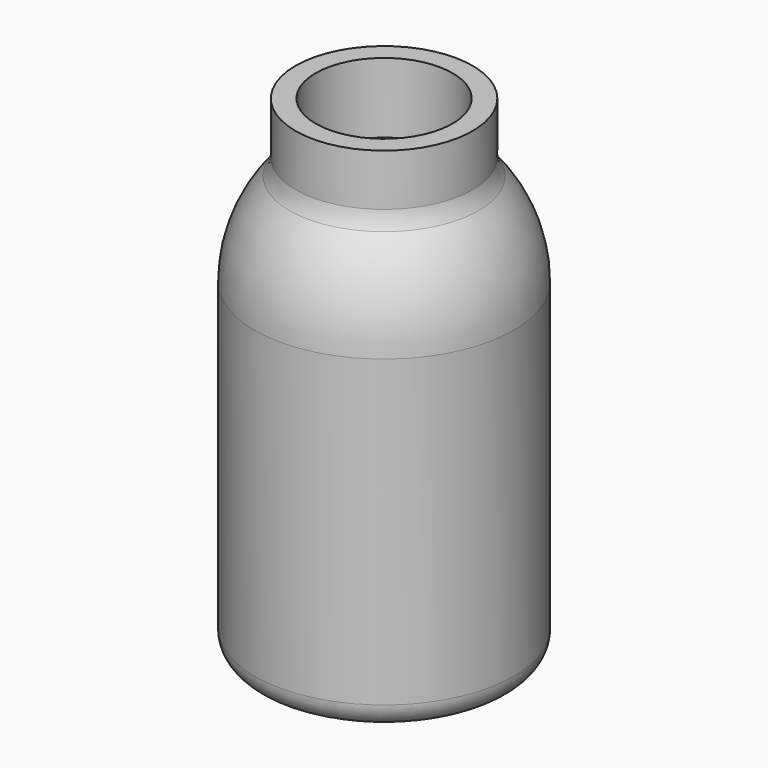
from build123d import *

# Parameters (mm, degrees)
F3_R = 5.08


# Not quite as in the source:
# - a fillet or chamfer that OpenCascade refuses, or shapes differently, is made with other operations: its cross-section is extruded or revolved along the edge and cut away or added


with BuildPart() as f1:
    # F0 (on Front) → F1 (revolve)
    with BuildSketch(Plane.XZ):
        with BuildLine():
            Line((-26.2792315334, 0), (-22.2152307564, 0))
            Line((-22.2152307564, 0), (-22.2152307564, 66.6416212916))
            ThreePointArc((-22.2152307564, 66.6416212916), (-20.0328257832, 76.8506354666), (-13.8671085173, 85.2750519145))
            Line((-13.8671085173, 85.2750519145), (-13.8671085173, 99.4861274958))
            Line((-13.8671085173, 99.4861274958), (-17.9311092943, 99.4861274958))
            Line((-17.9311092943, 99.4861274958), (-17.9311092943, 87.0146006346))
            ThreePointArc((-17.9311092943, 87.0146006346), (-24.1112579421, 77.6501342728), (-26.2792315334, 66.6416212916))
            Line((-26.2792315334, 66.6416212916), (-26.2792315334, 0))
        make_face()
    revolve(axis=Axis((0, 0, 49.7430637479), (0, 0, -1)))

    # F2: fillet of radius 5.08 on 1 edges, made by hand

    # F2_s1 → F2_t2 (revolve, cut)
    with BuildSketch(Plane.XZ):
        with BuildLine():
            ThreePointArc((-26.2796315334, 4.9781517325), (-25.134523883, 1.7647190024), (-22.2153108172, -0.0003919059))
            Line((-22.2153108172, -0.0003919059), (-22.3170153141, -0.4982462698))
            ThreePointArc((-22.3170153141, -0.4982462698), (-24.2472711753, -0.5081365685), (-26.2792315334, -0.5081365685))
            Line((-26.2792315334, -0.5081365685), (-26.787368102, 0))
            ThreePointArc((-26.787368102, 0), (-26.787368102, 2.4890758662), (-26.787768102, 4.9781517325))
            Line((-26.787768102, 4.9781517325), (-26.2796315334, 4.9781517325))
        make_face()
    revolve(axis=Axis((0, 0, 0), (0, 0, -1)), mode=Mode.SUBTRACT)

    # F3
    f3_edges = [f1.edges().sort_by_distance(p)[0] for p in [
        (17.931109, 0, 87.014601),
    ]]
    fillet(f3_edges, radius=F3_R)


solid = f1.part
